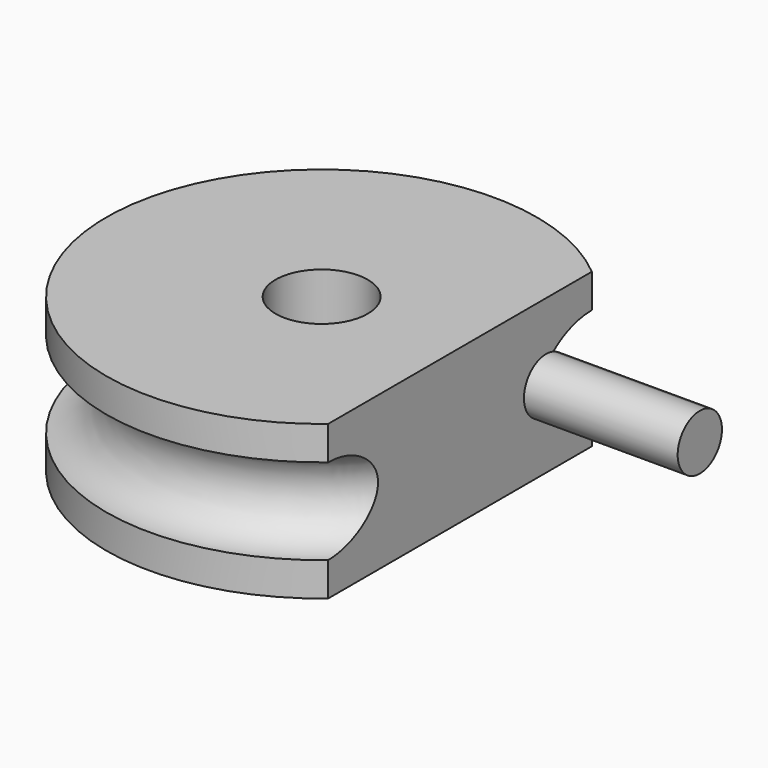
from build123d import *

# Parameters (mm, degrees)
F0_R     = 15
F1_DEPTH = 25
F5_DEPTH = 50


with BuildPart() as f1:
    # F0 (on Top) → F1 (new body, symmetric)
    with BuildSketch(Plane.XY):
        with BuildLine():
            Line((45, -53.6190264738), (45, 53.6190264738))
            ThreePointArc((45, 53.6190264738), (-70, 0), (45, -53.6190264738))
        make_face()
        Circle(F0_R, mode=Mode.SUBTRACT)
    extrude(amount=F1_DEPTH, both=True)

    # F2 (on Right) → F3 (revolve, cut)
    with BuildSketch(Plane.YZ):
        with BuildLine():
            Line((70, -14), (70, 14))
            ThreePointArc((70, 14), (56, 0), (70, -14))
        make_face()
    revolve(axis=Axis((0, 0, 25), (0, 0, 1)), mode=Mode.SUBTRACT)

    # F4 (on face) → F5 (join)
    with BuildSketch(Plane.YZ.offset(45)):
        with BuildLine():
            add(Edge.make_bspline(
                [(37.9630328609, 8.4982607788), (37.8523435019, 8.4048203415), (37.7424820724, 8.3104014762), (37.6334707776, 8.2149986154), (37.525332792, 8.1186060884), (37.4180922716, 8.0212181078), (37.3117743656, 7.9228287563), (37.2064052286, 7.823431974), (36.826236873, 7.4577676485), (36.5572934764, 7.185459665), (36.2956678052, 6.9059722624), (36.041930817, 6.6191996988), (35.7967338532, 6.3250596485), (35.5608040283, 6.0234970289), (35.3349396191, 5.7144878262), (34.9596041272, 5.1618860399), (34.8053000417, 4.9216027682), (34.6574566137, 4.677206923), (34.5164662374, 4.4287401627), (34.3827450871, 4.1762748231), (34.2567257621, 3.9199178725), (34.1388477747, 3.6598159897), (33.972823057, 3.2593369411), (33.9184105228, 3.1215569007), (33.8663694036, 2.9828498623), (33.8167604551, 2.8432475247), (33.769643447, 2.7027852726), (33.7250765475, 2.5615023849), (33.6831157079, 2.4194422423), (33.567344253, 1.998824599), (33.5009341193, 1.7182071188), (33.444986335, 1.43518271), (33.399847873, 1.1501662245), (33.3657973112, 0.8636063961), (33.3430321538, 0.5759874866), (33.331656153, 0.2878309318), (33.3316772398, -0.2920603513), (33.3433625212, -0.5838406442), (33.36672517, -0.8750615205), (33.4016558858, -1.1651818297), (33.4479469745, -1.4536998647), (33.5053059499, -1.7401515835), (33.5733691351, -2.024108832), (33.6915046183, -2.4479228858), (33.7339482932, -2.5899306957), (33.7789927091, -2.7311537294), (33.82658152, -2.8715490352), (33.8766562279, -3.0110777655), (33.9291567963, -3.1497049676), (33.984022265, -3.2873993744), (34.1490037446, -3.6819927579), (34.2650067533, -3.9364311557), (34.3887918355, -4.1872704013), (34.5199466609, -4.4343744462), (34.6580655419, -4.6776436303), (34.8027579562, -4.9170101221), (34.9536551707, -5.1524343498), (35.3248066319, -5.7004684421), (35.5501463092, -6.0096084062), (35.7855690187, -6.3113088937), (36.030274827, -6.6055929723), (36.2835351055, -6.8925150275), (36.5446977166, -7.1721564153), (36.8131911273, -7.4446219389), (37.1944947346, -7.8121861418), (37.3014725192, -7.9132878967), (37.409432192, -8.0133489318), (37.5183462275, -8.1123756019), (37.6281881757, -8.2103741117), (37.7389326494, -8.3073505305), (37.8505553113, -8.403310806), (37.9630328615, -8.4982607786)],
                knots=[0.3142800556, 0.3142800556, 0.3142800556, 0.3142800556, 0.3142800556, 0.3142800556, 0.3142800556, 0.3142800556, 0.3142800556, 0.3358087351, 0.3358087351, 0.3358087351, 0.3358087351, 0.3358087351, 0.3358087351, 0.3358087351, 0.3926809759, 0.3926809759, 0.3926809759, 0.3926809759, 0.3926809759, 0.3926809759, 0.3926809759, 0.43512366, 0.43512366, 0.43512366, 0.43512366, 0.43512366, 0.43512366, 0.43512366, 0.4571495261, 0.4571495261, 0.4571495261, 0.4571495261, 0.4571495261, 0.4571495261, 0.4571495261, 0.5000055628, 0.5000055628, 0.5000055628, 0.5000055628, 0.5000055628, 0.5000055628, 0.5000055628, 0.5434005305, 0.5434005305, 0.5434005305, 0.5434005305, 0.5434005305, 0.5434005305, 0.5434005305, 0.5654393693, 0.5654393693, 0.5654393693, 0.5654393693, 0.5654393693, 0.5654393693, 0.5654393693, 0.6070013278, 0.6070013278, 0.6070013278, 0.6070013278, 0.6070013278, 0.6070013278, 0.6070013278, 0.6638433094, 0.6638433094, 0.6638433094, 0.6638433094, 0.6638433094, 0.6638433094, 0.6638433094, 0.6857197919, 0.6857197919, 0.6857197919, 0.6857197919, 0.6857197919, 0.6857197919, 0.6857197919, 0.6857197919, 0.6857197919], degree=8))
            ThreePointArc((37.9630328609, 8.4982607788), (26, -3e-10), (37.9630328615, -8.4982607786))
        make_face()
        with BuildLine():
            ThreePointArc((37.9630328615, -8.4982607786), (42.3371416694, -5.212135083), (44, 0))
            ThreePointArc((44, 0), (42.3371416692, 5.2121350832), (37.9630328609, 8.4982607788))
            add(Edge.make_bspline(
                [(37.9630328609, 8.4982607788), (37.8523435019, 8.4048203415), (37.7424820724, 8.3104014762), (37.6334707776, 8.2149986154), (37.525332792, 8.1186060884), (37.4180922716, 8.0212181078), (37.3117743656, 7.9228287563), (37.2064052286, 7.823431974), (36.826236873, 7.4577676485), (36.5572934764, 7.185459665), (36.2956678052, 6.9059722624), (36.041930817, 6.6191996988), (35.7967338532, 6.3250596485), (35.5608040283, 6.0234970289), (35.3349396191, 5.7144878262), (34.9596041272, 5.1618860399), (34.8053000417, 4.9216027682), (34.6574566137, 4.677206923), (34.5164662374, 4.4287401627), (34.3827450871, 4.1762748231), (34.2567257621, 3.9199178725), (34.1388477747, 3.6598159897), (33.972823057, 3.2593369411), (33.9184105228, 3.1215569007), (33.8663694036, 2.9828498623), (33.8167604551, 2.8432475247), (33.769643447, 2.7027852726), (33.7250765475, 2.5615023849), (33.6831157079, 2.4194422423), (33.567344253, 1.998824599), (33.5009341193, 1.7182071188), (33.444986335, 1.43518271), (33.399847873, 1.1501662245), (33.3657973112, 0.8636063961), (33.3430321538, 0.5759874866), (33.331656153, 0.2878309318), (33.3316772398, -0.2920603513), (33.3433625212, -0.5838406442), (33.36672517, -0.8750615205), (33.4016558858, -1.1651818297), (33.4479469745, -1.4536998647), (33.5053059499, -1.7401515835), (33.5733691351, -2.024108832), (33.6915046183, -2.4479228858), (33.7339482932, -2.5899306957), (33.7789927091, -2.7311537294), (33.82658152, -2.8715490352), (33.8766562279, -3.0110777655), (33.9291567963, -3.1497049676), (33.984022265, -3.2873993744), (34.1490037446, -3.6819927579), (34.2650067533, -3.9364311557), (34.3887918355, -4.1872704013), (34.5199466609, -4.4343744462), (34.6580655419, -4.6776436303), (34.8027579562, -4.9170101221), (34.9536551707, -5.1524343498), (35.3248066319, -5.7004684421), (35.5501463092, -6.0096084062), (35.7855690187, -6.3113088937), (36.030274827, -6.6055929723), (36.2835351055, -6.8925150275), (36.5446977166, -7.1721564153), (36.8131911273, -7.4446219389), (37.1944947346, -7.8121861418), (37.3014725192, -7.9132878967), (37.409432192, -8.0133489318), (37.5183462275, -8.1123756019), (37.6281881757, -8.2103741117), (37.7389326494, -8.3073505305), (37.8505553113, -8.403310806), (37.9630328615, -8.4982607786)],
                knots=[0.3142800556, 0.3142800556, 0.3142800556, 0.3142800556, 0.3142800556, 0.3142800556, 0.3142800556, 0.3142800556, 0.3142800556, 0.3358087351, 0.3358087351, 0.3358087351, 0.3358087351, 0.3358087351, 0.3358087351, 0.3358087351, 0.3926809759, 0.3926809759, 0.3926809759, 0.3926809759, 0.3926809759, 0.3926809759, 0.3926809759, 0.43512366, 0.43512366, 0.43512366, 0.43512366, 0.43512366, 0.43512366, 0.43512366, 0.4571495261, 0.4571495261, 0.4571495261, 0.4571495261, 0.4571495261, 0.4571495261, 0.4571495261, 0.5000055628, 0.5000055628, 0.5000055628, 0.5000055628, 0.5000055628, 0.5000055628, 0.5000055628, 0.5434005305, 0.5434005305, 0.5434005305, 0.5434005305, 0.5434005305, 0.5434005305, 0.5434005305, 0.5654393693, 0.5654393693, 0.5654393693, 0.5654393693, 0.5654393693, 0.5654393693, 0.5654393693, 0.6070013278, 0.6070013278, 0.6070013278, 0.6070013278, 0.6070013278, 0.6070013278, 0.6070013278, 0.6638433094, 0.6638433094, 0.6638433094, 0.6638433094, 0.6638433094, 0.6638433094, 0.6638433094, 0.6857197919, 0.6857197919, 0.6857197919, 0.6857197919, 0.6857197919, 0.6857197919, 0.6857197919, 0.6857197919, 0.6857197919], degree=8))
        make_face()
    extrude(amount=F5_DEPTH)


solid = f1.part
